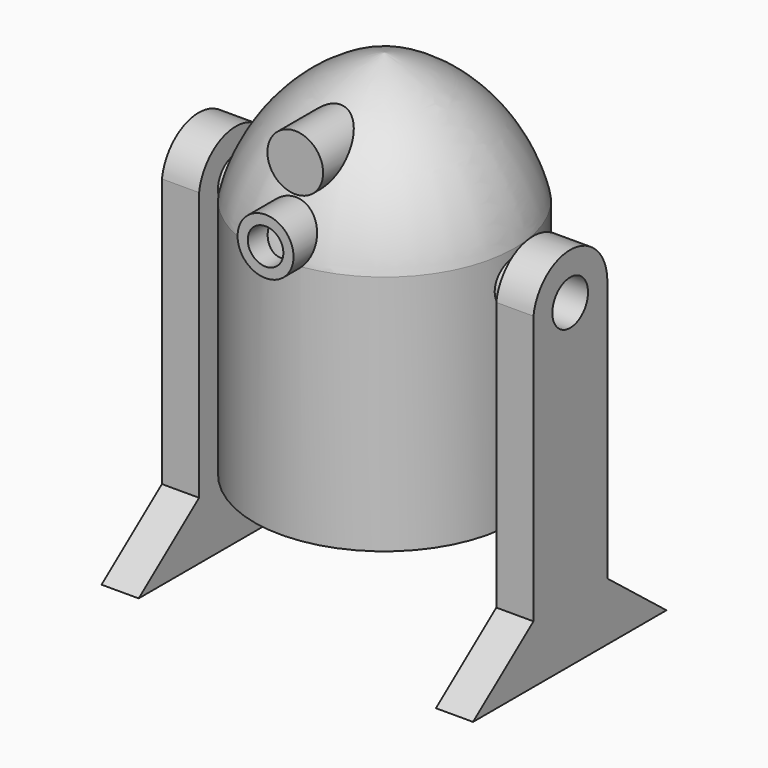
from build123d import *

# Parameters (mm, degrees)
F2_R     = 6
F3_DEPTH = 40
F4_R     = 6
F5_DEPTH = 10
F6_R     = 7.5
F7_DEPTH = 30
F8_R     = 7.5344218683
F8_R_2   = 4.7967964391
F9_DEPTH = 40


# Not quite as in the source:
# - a pattern or mirror of a feature is missing from the dataset's text; its kind, count and spacing are read off the source's solid


with BuildPart() as f1:
    # F0 (on Front) → F1 (revolve)
    with BuildSketch(Plane.XZ):
        with BuildLine():
            Line((0, 100), (0, 0))
            Line((0, 0), (35, 0))
            Line((35, 0), (35, 65))
            ThreePointArc((35, 65), (22.3890116119, 87.3890116119), (0, 100))
        make_face()
    revolve(axis=Axis((0, 0, 50), (0, 0, 1)))

    # F2 (on Right) → F3 (join)
    with BuildSketch(Plane.YZ):
        with Locations((0, 57)):
            Circle(F2_R)
    f3 = extrude(amount=F3_DEPTH)

    # F3_copies: F3 across plane
    add(f3.mirror(Plane(origin=(0, 0, 0), x_dir=(0, 0, -1), z_dir=(-1, 0, 0))))

    # F6 (on Front) → F7 (join)
    with BuildSketch(Plane.XZ):
        with Locations((0, 86.1279029752)):
            Circle(F6_R)
    extrude(amount=F7_DEPTH)

    # F8 (on Front) → F9 (join)
    with BuildSketch(Plane.XZ):
        with Locations((0, 70.3167021275)):
            Circle(F8_R)
        with Locations((0, 70.3167021275)):
            Circle(F8_R_2, mode=Mode.SUBTRACT)
    extrude(amount=F9_DEPTH)


with BuildPart() as f5:
    # F4 (on face) → F5 (new body)
    with BuildSketch(Plane.YZ.offset(40)):
        with BuildLine():
            Line((12.4931683911, -13.4557196397), (12.4931683911, 56.5867887339))
            Line((12.4931683911, 56.5867887339), (12.4931683911, 57.4132112661))
            ThreePointArc((12.4931683911, 57.4132112661), (0.7114896822, 69.4797348703), (-12.3652548185, 58.8304298058))
            Line((-12.3652548185, 58.8304298058), (-12.3652548185, 55.1695701942))
            Line((-12.3652548185, 55.1695701942), (-12.3652548185, -13.4957142435))
            Line((-12.3652548185, -13.4957142435), (-32.6849780977, -29.0772188455))
            Line((-32.6849780977, -29.0772188455), (-17.0291475952, -29.0772188455))
            Line((-17.0291475952, -29.0772188455), (32.3974410422, -29.0772188455))
            Line((32.3974410422, -29.0772188455), (12.4931683911, -13.4557196397))
        make_face()
        with Locations((0, 57)):
            Circle(F4_R, mode=Mode.SUBTRACT)
    extrude(amount=F5_DEPTH)


with BuildPart() as f5_copies_1:
    # F5_copies: instance of F5
    add(f5.part.mirror(Plane(origin=(0, 0, 0), x_dir=(0, 0, -1), z_dir=(-1, 0, 0))))


solid = Compound([f1.part, f5.part, f5_copies_1.part])
